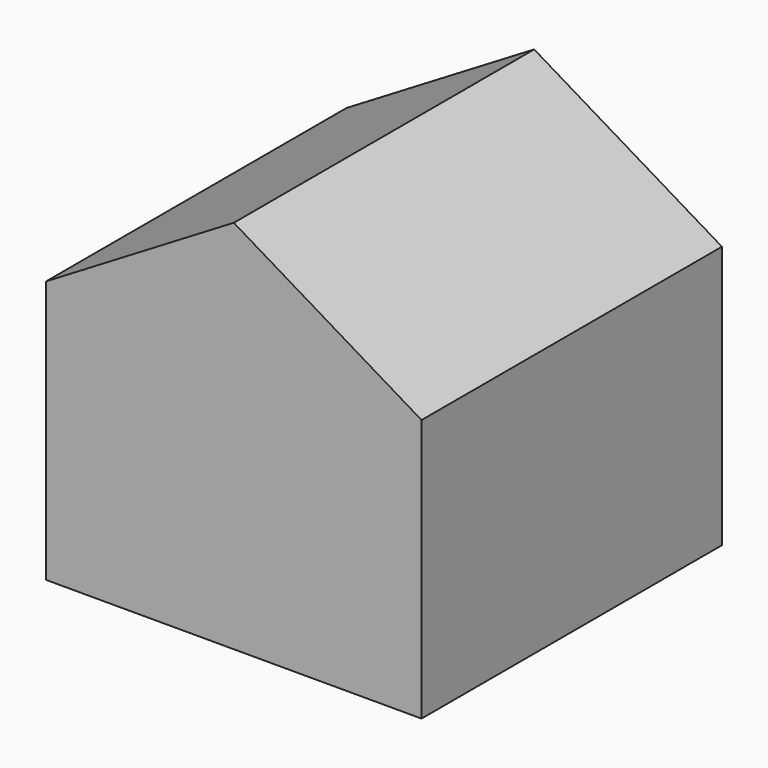
from build123d import *

# Parameters (mm, degrees)
F0_W     = 50
F0_H     = 50
F0_W_2   = 40
F0_H_2   = 40
F1_DEPTH = 25
F2_W     = 50
F2_H     = 50
F3_DEPTH = 25
F4_SIZE2 = 14.99999
F4_SIZE  = 24.99999


# Not quite as in the source:
# - a fillet or chamfer is up to 0.001 mm smaller than in the source, because OpenCascade refuses the exact size


with BuildPart() as f1:
    # F0 (on Top) → F1 (new body)
    with BuildSketch(Plane.XY):
        with Locations((-34.6303719711, 27.0920880139)):
            Rectangle(F0_W, F0_H)
        with Locations((-34.6303719711, 27.0920880139)):
            Rectangle(F0_W_2, F0_H_2, mode=Mode.SUBTRACT)
    extrude(amount=F1_DEPTH)

    # F2 (on face) → F3 (join)
    with BuildSketch(Plane.XY.offset(25)):
        with Locations((-34.6303719711, 27.0920880139)):
            Rectangle(F2_W, F2_H)
    extrude(amount=F3_DEPTH)

    # F4 (size 25 and 15 in the source; OpenCascade refuses exactly that, so slightly less here)
    f4_edges = [f1.edges().sort_by_distance(p)[0] for p in [
        (-59.630372, 27.092088, 50),
        (-9.630372, 27.092088, 50),
    ]]
    f4_side = f1.faces().sort_by_distance((-34.630372, 27.092088, 50))[0]
    chamfer(f4_edges, length=F4_SIZE, length2=F4_SIZE2, reference=f4_side)


solid = f1.part
